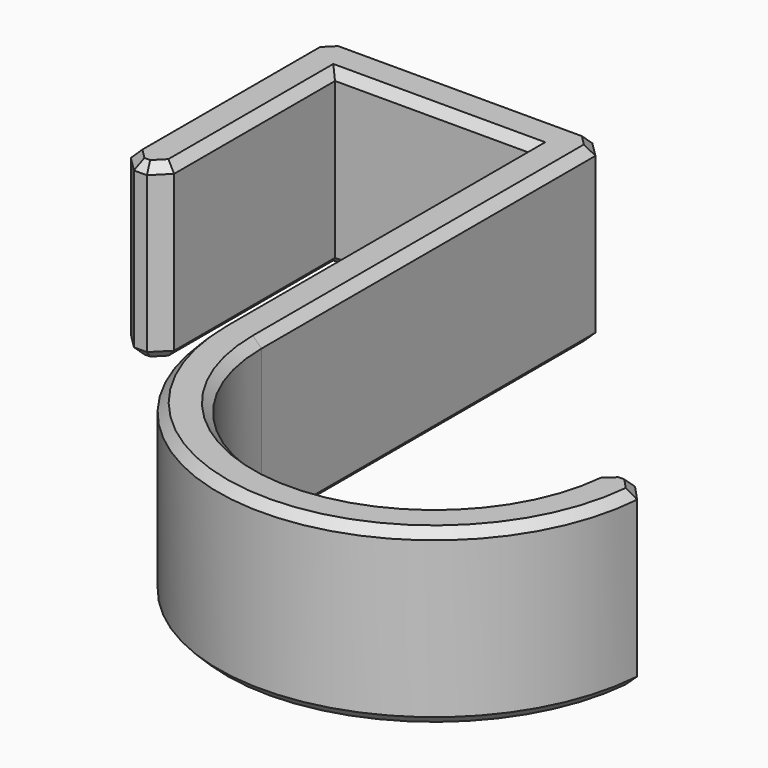
from build123d import *

# Parameters (mm, degrees)
F1_DEPTH    = 8
F2_T1_DEPTH = 11.6003561832
F2_T3_DEPTH = 11.8663751546
F2_T5_DEPTH = 11.4631685347
F3_SIZE     = 0.4


# Not quite as in the source:
# - a fillet or chamfer that OpenCascade refuses, or shapes differently, is made with other operations: its cross-section is extruded or revolved along the edge and cut away or added


with BuildPart() as f1:
    # F0 (on Top) → F1 (new body)
    with BuildSketch(Plane.XY):
        with BuildLine():
            Line((-21, 8), (-19, 8))
            Line((-19, 8), (-19, 18))
            Line((-19, 18), (-10, 18))
            Line((-10, 18), (-10, 0))
            ThreePointArc((-10, 0), (0, -10), (10, 0))
            Line((10, 0), (8, 0))
            ThreePointArc((8, 0), (0, -8), (-8, 0))
            Line((-8, 0), (-8, 20))
            Line((-8, 20), (-21, 20))
            Line((-21, 20), (-21, 8))
        make_face()
    extrude(amount=F1_DEPTH)

    # F2: chamfer of 0.7 on 6 edges, made by hand

    # F2_s2 → F2_t1 (cut)
    with BuildSketch(Plane.XY.offset(-1.8001780916)):
        Polygon((-8, 19.3), (-8.7, 20), (-8, 20), align=None)
        Polygon((-20.3, 20), (-21, 19.3), (-21, 20), align=None)
        Polygon((-20.3, 8), (-21, 8.7), (-21, 8), align=None)
        Polygon((-19.7, 8), (-19, 8.7), (-19, 8), align=None)
    extrude(amount=F2_T1_DEPTH, mode=Mode.SUBTRACT)

    # F2_s4 → F2_t3 (cut)
    with BuildSketch(Plane.XY.offset(-1.9331875773)):
        with BuildLine():
            Line((9.9716327909, -0.752688172), (9.2736184955, 0))
            Line((9.2736184955, 0), (10, 0))
            ThreePointArc((10, 0), (9.9925280661, -0.3865007745), (9.9716327909, -0.752688172))
        make_face()
    extrude(amount=F2_T3_DEPTH, mode=Mode.SUBTRACT)

    # F2_s6 → F2_t5 (cut)
    with BuildSketch(Plane.XY.offset(-1.7315842673)):
        with BuildLine():
            Line((8.6717933555, 0), (7.9740628556, -0.6436781609))
            ThreePointArc((7.9740628556, -0.6436781609), (7.9931075422, -0.332011775), (8, 0))
            Line((8, 0), (8.6717933555, 0))
        make_face()
    extrude(amount=F2_T5_DEPTH, mode=Mode.SUBTRACT)

    # F3
    f3_edges = [f1.edges().sort_by_distance(p)[0] for p in [
        (-20.65, 19.65, 8),
        (-14.5, 20, 8),
        (-8.35, 19.65, 8),
        (-8, 9.65, 8),
        (-0.3221, -7.993513, 8),
        (8.322928, -0.321839, 8),
        (8.972706, 0, 8),
        (9.622626, -0.376344, 8),
        (-0.376611, -9.992906, 8),
        (-10, 9, 8),
        (-14.5, 18, 8),
        (-19, 13.35, 8),
        (-19.35, 8.35, 8),
        (-20, 8, 8),
        (-20.65, 8.35, 8),
        (-21, 14, 8),
        (-20.65, 19.65, 0),
        (-14.5, 20, 0),
        (-8.35, 19.65, 0),
        (-8, 9.65, 0),
        (-0.3221, -7.993513, 0),
        (8.322928, -0.321839, 0),
        (8.972706, 0, 0),
        (9.622626, -0.376344, 0),
        (-0.376611, -9.992906, 0),
        (-10, 9, 0),
        (-14.5, 18, 0),
        (-19, 13.35, 0),
        (-19.35, 8.35, 0),
        (-20, 8, 0),
        (-20.65, 8.35, 0),
        (-21, 14, 0),
    ]]
    chamfer(f3_edges, length=F3_SIZE)


solid = f1.part
